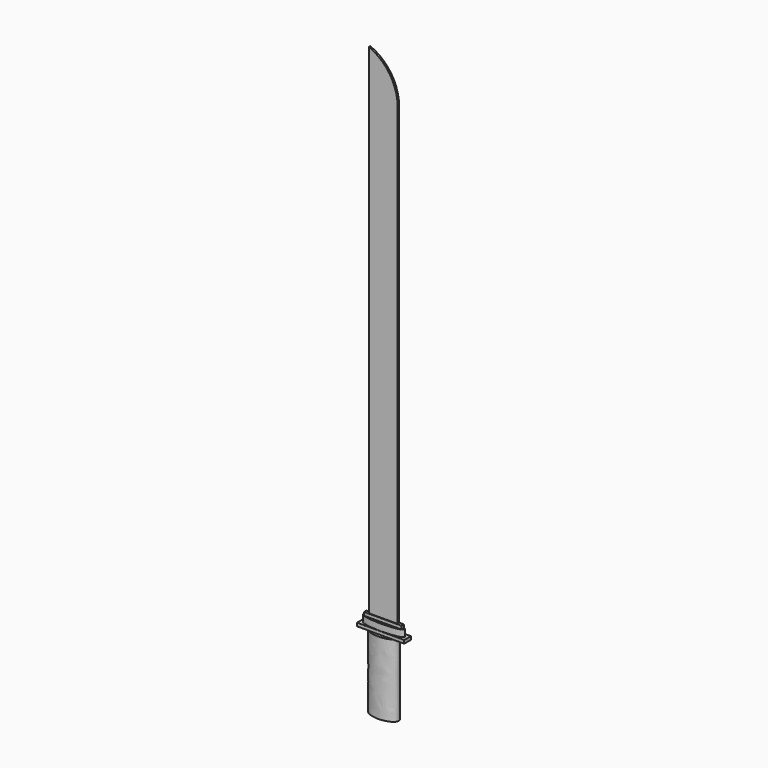
from build123d import *

# Parameters (mm, degrees)
F0_W        = 217.7935391665
F0_H        = 13.5906832293
F1_DEPTH    = 3780
F2_T1_DEPTH = 1658.3004497915
F3_W        = 284.022539854
F3_H        = 23.1398101896
F4_DEPTH    = 25
F7_DEPTH    = 50
F9_W        = 357.4613034725
F9_H        = 63.879750669
F10_DEPTH   = 25
F13_DEPTH   = 550


# Not quite as in the source:
# - a fillet or chamfer that OpenCascade refuses, or shapes differently, is made with other operations: its cross-section is extruded or revolved along the edge and cut away or added


with BuildPart() as f1:
    # F0 (on Top) → F1 (new body)
    with BuildSketch(Plane.XY):
        Rectangle(F0_W, F0_H)
    extrude(amount=F1_DEPTH)

    # F2: fillet of radius 357.3036072312 on 1 edges, made by hand

    # F2_s2 → F2_t1 (cut)
    with BuildSketch(Plane.XZ.offset(-829.1502248957)):
        with BuildLine():
            ThreePointArc((108.8967695832, 3451.0580466876), (49.513720811, 3648.3122192364), (-108.8967695832, 3780))
            Line((-108.8967695832, 3780), (108.8967695832, 3780))
            Line((108.8967695832, 3780), (108.8967695832, 3451.0580466876))
        make_face()
    extrude(amount=F2_T1_DEPTH, mode=Mode.SUBTRACT)

    # F3 (on Top) → F4 (join)
    with BuildSketch(Plane.XY):
        Rectangle(F3_W, F3_H)
    extrude(amount=-F4_DEPTH)

    # F6 (on offset) → F7 (join)
    with BuildSketch(Plane.XY.offset(-25)):
        with BuildLine():
            add(Edge.make_bspline(
                [(157.1267843246, 0), (157.1267843246, 51.8759819398), (-78.5633921623, 25.9379909699), (-314.2535686493, 0), (-78.5633921623, -25.9379909699), (157.1267843246, -51.8759819398), (157.1267843246, 0)],
                knots=[0, 0, 0, 2.0943951024, 2.0943951024, 4.1887902048, 4.1887902048, 6.2831853072, 6.2831853072, 6.2831853072], degree=2, weights=[1, 0.5, 1, 0.5, 1, 0.5, 1]))
        make_face()
    extrude(amount=-F7_DEPTH)

    # F9 (on offset) → F10 (join)
    with BuildSketch(Plane.XY.offset(-75)):
        Rectangle(F9_W, F9_H)
    extrude(amount=-F10_DEPTH)

    # F12 (on offset) → F13 (join)
    with BuildSketch(Plane.XY.offset(-100)):
        with BuildLine():
            add(Edge.make_bspline(
                [(111.7473468184, 0), (111.7473468184, 96.4192818942), (-55.8736734092, 48.2096409471), (-223.4946936369, 0), (-55.8736734092, -48.2096409471), (111.7473468184, -96.4192818942), (111.7473468184, 0)],
                knots=[0, 0, 0, 2.0943951024, 2.0943951024, 4.1887902048, 4.1887902048, 6.2831853072, 6.2831853072, 6.2831853072], degree=2, weights=[1, 0.5, 1, 0.5, 1, 0.5, 1]))
        make_face()
    extrude(amount=-F13_DEPTH)


solid = f1.part
